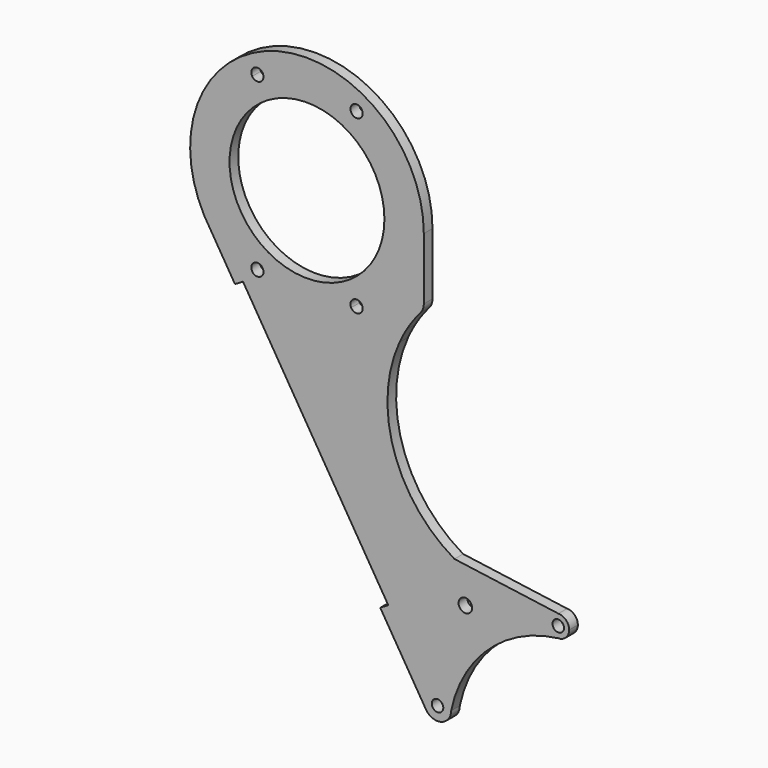
from build123d import *

# Parameters (mm, degrees)
F0_R     = 4.25
F0_R_2   = 57
F1_DEPTH = 8


# Not quite as in the source:
# - a feature names something its author has since deleted; it is built from what else it names


with BuildPart() as f1:
    # F0 (on Front) → F1 (new body)
    with BuildSketch(Plane.XZ):
        with BuildLine():
            Line((86, -45.5504168361), (86, 0))
            ThreePointArc((86, 0), (25.52491441, -82.1247754601), (-70.8483428922, -48.7494852222))
            Line((-70.8483428922, -48.7494852222), (-52.9901534319, -77.9586575178))
            Line((-52.9901534319, -77.9586575178), (-47.1157296051, -74.3670948194))
            Line((-47.1157296051, -74.3670948194), (59.817007023, -249.2681806857))
            Line((59.817007023, -249.2681806857), (53.9425831962, -252.8597433842))
            Line((53.9425831962, -252.8597433842), (87.570656583, -307.862418303))
            ThreePointArc((87.570656583, -307.862418303), (86.7439526122, -299.1221062681), (93.1304247757, -293.0980322955))
            ThreePointArc((93.1304247757, -293.0980322955), (102.0303203377, -294.5926190657), (106.1024168691, -302.646187248))
            ThreePointArc((106.1024168691, -302.646187248), (106.1023341619, -302.6868583365), (106.1020860416, -302.7275287523))
            ThreePointArc((106.1020860416, -302.7275287523), (133.8669990345, -253.7041794438), (184.9928569387, -230.0329770139))
            ThreePointArc((184.9928569387, -230.0329770139), (176.9929095406, -222.0039661985), (185.0508781881, -214.0331874208))
            Line((185.0508781881, -214.0331874208), (108.5283892756, -203.5204235365))
            ThreePointArc((108.5283892756, -203.5204235365), (63.9114156279, -147.6449683437), (68.1014852993, -76.2644097396))
            ThreePointArc((68.1014852993, -76.2644097396), (70.6109477759, -71.1161938658), (73.4114917534, -66.1203473875))
            ThreePointArc((73.4114917534, -66.1203473875), (78.1822601822, -58.8864182021), (83.5623402825, -52.0934290975))
            ThreePointArc((83.5623402825, -52.0934290975), (85.3707897966, -49.0415912213), (86, -45.5504168361))
        make_face()
        with BuildLine():
            ThreePointArc((116.5832400171, -226.0398806244), (120.1187739231, -227.5043467184), (121.5832400171, -231.0398806244))
            ThreePointArc((121.5832400171, -231.0398806244), (113.0477061112, -234.5754145303), (116.5832400171, -226.0398806244))
        make_face(mode=Mode.SUBTRACT)
        with BuildLine():
            ThreePointArc((93.1304247757, -293.0980322955), (86.7439526122, -299.1221062681), (87.570656583, -307.862418303))
            ThreePointArc((87.570656583, -307.862418303), (98.7727093249, -312.2830715059), (106.1020860416, -302.7275287523))
            ThreePointArc((106.1020860416, -302.7275287523), (106.1023341619, -302.6868583365), (106.1024168691, -302.646187248))
            ThreePointArc((106.1024168691, -302.646187248), (102.0303203377, -294.5926190657), (93.1304247757, -293.0980322955))
        make_face()
        with BuildLine():
            ThreePointArc((100.3524168691, -302.646187248), (93.583057895, -306.0689537255), (94.8393202294, -298.5882213932))
            ThreePointArc((94.8393202294, -298.5882213932), (98.6217758433, -299.2234207705), (100.3524168691, -302.646187248))
        make_face(mode=Mode.SUBTRACT)
        with BuildLine():
            ThreePointArc((192.9928569387, -222.0329770139), (190.6701877373, -216.3966737039), (185.0508781881, -214.0331874208))
            ThreePointArc((185.0508781881, -214.0331874208), (176.9929095406, -222.0039661985), (184.9928569387, -230.0329770139))
            ThreePointArc((184.9928569387, -230.0329770139), (190.6497111882, -227.6898312634), (192.9928569387, -222.0329770139))
        make_face()
        with Locations((184.9928569387, -222.0329770139)):
            Circle(F0_R, mode=Mode.SUBTRACT)
        with BuildLine():
            ThreePointArc((-70.8483428922, -48.7494852222), (25.52491441, -82.1247754601), (86, 0))
            ThreePointArc((86, 0), (-21.0609353072, 83.3812749002), (-75.6845814881, -40.8392473605))
            Line((-75.6845814881, -40.8392473605), (-70.8483428922, -48.7494852222))
        make_face()
        with BuildLine():
            ThreePointArc((40.3259134511, 60.8508069325), (64.3148182067, 34.5341013932), (73, 0))
            ThreePointArc((73, 0), (64.3148182067, -34.5341013932), (40.3259134511, -60.8508069325))
            ThreePointArc((40.3259134511, -60.8508069325), (40.8281988477, -61.9883128671), (41, -63.2198544763))
            ThreePointArc((41, -63.2198544763), (37.5975531045, -67.5839554355), (32.5353879188, -65.3486689457))
            ThreePointArc((32.5353879188, -65.3486689457), (0, -73), (-32.5353879188, -65.3486689457))
            ThreePointArc((-32.5353879188, -65.3486689457), (-38.75, -67.1169687933), (-40.3259134511, -60.8508069325))
            ThreePointArc((-40.3259134511, -60.8508069325), (-73, 0), (-40.3259134511, 60.8508069325))
            ThreePointArc((-40.3259134511, 60.8508069325), (-38.75, 67.1169687933), (-32.5353879188, 65.3486689457))
            ThreePointArc((-32.5353879188, 65.3486689457), (0, 73), (32.5353879188, 65.3486689457))
            ThreePointArc((32.5353879188, 65.3486689457), (37.5975531045, 67.5839554355), (41, 63.2198544763))
            ThreePointArc((41, 63.2198544763), (40.8281988477, 61.9883128671), (40.3259134511, 60.8508069325))
        make_face(mode=Mode.SUBTRACT)
        with BuildLine():
            ThreePointArc((40.3259134511, -60.8508069325), (64.3148182067, -34.5341013932), (73, 0))
            ThreePointArc((73, 0), (64.3148182067, 34.5341013932), (40.3259134511, 60.8508069325))
            ThreePointArc((40.3259134511, 60.8508069325), (34.25, 59.3227401592), (32.5353879188, 65.3486689457))
            ThreePointArc((32.5353879188, 65.3486689457), (0, 73), (-32.5353879188, 65.3486689457))
            ThreePointArc((-32.5353879188, 65.3486689457), (-32.1358990407, 64.3174075808), (-32, 63.2198544763))
            ThreePointArc((-32, 63.2198544763), (-35.2684583909, 58.8916556286), (-40.3259134511, 60.8508069325))
            ThreePointArc((-40.3259134511, 60.8508069325), (-73, 0), (-40.3259134511, -60.8508069325))
            ThreePointArc((-40.3259134511, -60.8508069325), (-35.2684583909, -58.8916556286), (-32, -63.2198544763))
            ThreePointArc((-32, -63.2198544763), (-32.1358990407, -64.3174075808), (-32.5353879188, -65.3486689457))
            ThreePointArc((-32.5353879188, -65.3486689457), (0, -73), (32.5353879188, -65.3486689457))
            ThreePointArc((32.5353879188, -65.3486689457), (34.25, -59.3227401592), (40.3259134511, -60.8508069325))
        make_face()
        Circle(F0_R_2, mode=Mode.SUBTRACT)
    extrude(amount=F1_DEPTH)


solid = f1.part
